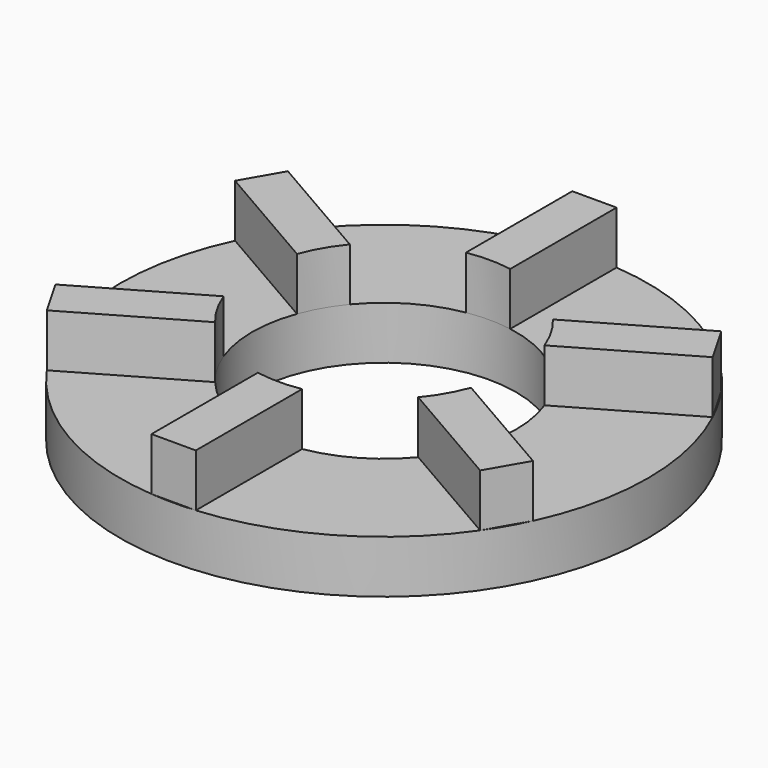
from build123d import *

# Parameters (mm, degrees)
F0_R     = 5
F0_R_2   = 2.5
F1_DEPTH = 1
F3_DEPTH = 1


# Not quite as in the source:
# - after a boolean that leaves OpenCascade's solid faulty, fix() repairs it


with BuildPart() as f1:
    # F0 (on Top) → F1 (new body)
    with BuildSketch(Plane.XY):
        Circle(F0_R)
        Circle(F0_R_2, mode=Mode.SUBTRACT)
    extrude(amount=F1_DEPTH)

    # F2 (on face) → F3 (join)
    with BuildSketch(Plane.XY.offset(1)):
        with BuildLine():
            ThreePointArc((-0.4197226159, 2.4645147445), (0, 2.5), (0.4197226159, 2.4645147445))
            Line((0.4197226159, 2.4645147445), (0.4197226159, 4.9823521479))
            Line((0.4197226159, 4.9823521479), (-0.4197226159, 4.9823521479))
            Line((-0.4197226159, 4.9823521479), (-0.4197226159, 2.4645147445))
        make_face()
        with BuildLine():
            ThreePointArc((-2.3441936847, 0.8687669243), (-2.1650635095, 1.25), (-1.9244710687, 1.5957478202))
            Line((-1.9244710687, 1.5957478202), (-4.1049822227, 2.8546665219))
            Line((-4.1049822227, 2.8546665219), (-4.5247048387, 2.127685626))
            Line((-4.5247048387, 2.127685626), (-2.3441936847, 0.8687669243))
        make_face()
        with BuildLine():
            ThreePointArc((-1.9244710687, -1.5957478202), (-2.1650635095, -1.25), (-2.3441936847, -0.8687669243))
            Line((-2.3441936847, -0.8687669243), (-4.5247048387, -2.127685626))
            Line((-4.5247048387, -2.127685626), (-4.1049822227, -2.8546665219))
            Line((-4.1049822227, -2.8546665219), (-1.9244710687, -1.5957478202))
        make_face()
        with BuildLine():
            ThreePointArc((0.4197226159, -2.4645147445), (0, -2.5), (-0.4197226159, -2.4645147445))
            Line((-0.4197226159, -2.4645147445), (-0.4197226159, -4.9823521479))
            Line((-0.4197226159, -4.9823521479), (0.4197226159, -4.9823521479))
            Line((0.4197226159, -4.9823521479), (0.4197226159, -2.4645147445))
        make_face()
        with BuildLine():
            Line((4.5247048387, -2.127685626), (2.3441936847, -0.8687669243))
            ThreePointArc((2.3441936847, -0.8687669243), (2.1650635095, -1.25), (1.9244710687, -1.5957478202))
            Line((1.9244710687, -1.5957478202), (4.1049822227, -2.8546665219))
            Line((4.1049822227, -2.8546665219), (4.5247048387, -2.127685626))
        make_face()
        with BuildLine():
            Line((4.1049822227, 2.8546665219), (1.9244710687, 1.5957478202))
            ThreePointArc((1.9244710687, 1.5957478202), (2.1650635095, 1.25), (2.3441936847, 0.8687669243))
            Line((2.3441936847, 0.8687669243), (4.5247048387, 2.127685626))
            Line((4.5247048387, 2.127685626), (4.1049822227, 2.8546665219))
        make_face()
    extrude(amount=F3_DEPTH)

    add(f1.part.fix(), mode=Mode.REPLACE)


solid = f1.part
